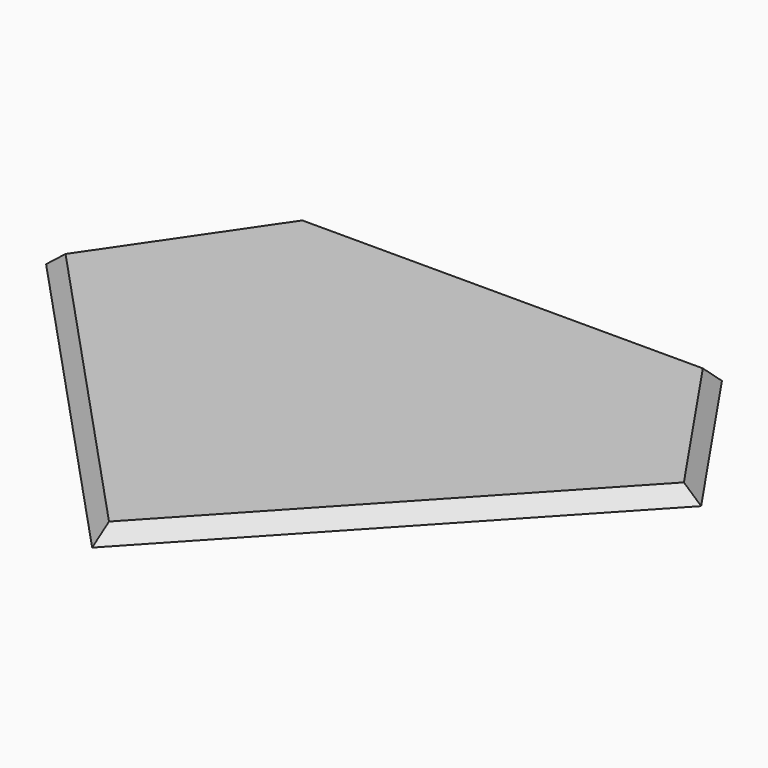
from build123d import *

# Parameters (mm, degrees)
F1_DEPTH    = 2.4268273264
F2_T1_DEPTH = 99.1532575298
F3_T1_DEPTH = 59.396472342
F4_T1_DEPTH = 59.396472342
F5_T1_DEPTH = 107.0840707021
F6_T1_DEPTH = 101.9910508867


# Not quite as in the source:
# - a fillet or chamfer that OpenCascade refuses, or shapes differently, is made with other operations: its cross-section is extruded or revolved along the edge and cut away or added


with BuildPart() as f1:
    # F0 (on Top) → F1 (new body)
    with BuildSketch(Plane.XY):
        Polygon((0, 32.5707793236), (-36.5124791861, 32.5707793236), (-58.7103962898, 0), (0, -63.0669593811), align=None)
        Polygon((36.5124791861, 32.5707793236), (0, 32.5707793236), (0, -63.0669593811), (58.7103962898, 0), align=None)
    extrude(amount=F1_DEPTH)

    # F2: chamfer of 5.08 on 1 edges, made by hand

    # F2_s2 → F2_t1 (cut)
    with BuildSketch(Plane.YZ.offset(-49.5766287649)):
        Polygon((32.5707793236, -2.6531726736), (27.4907793236, 2.4268273264), (32.5707793236, 2.4268273264), align=None)
    extrude(amount=F2_T1_DEPTH, mode=Mode.SUBTRACT)

    # F3: chamfer of 5.08 on 1 edges, made by hand

    # F3_s2 → F3_t1 (cut)
    with BuildSketch(Plane(origin=(7.4722902543, 10.964015938, 0), x_dir=(0, 0, 1), z_dir=(-0.5631734509, -0.8263387103, 0))):
        Polygon((-2.6531726736, 48.5146731522), (2.4268273264, 43.4346731522), (2.4268273264, 48.5146731522), align=None)
    extrude(amount=F3_T1_DEPTH, mode=Mode.SUBTRACT)

    # F4: chamfer of 5.08 on 1 edges, made by hand

    # F4_s2 → F4_t1 (cut)
    with BuildSketch(Plane(origin=(25.9782260477, -38.1175884143, 0), x_dir=(0, 0, 1), z_dir=(-0.5631734509, 0.8263387103, 0))):
        Polygon((-2.6531726736, 48.5146731522), (2.4268273264, 43.4346731522), (2.4268273264, 48.5146731522), align=None)
    extrude(amount=F4_T1_DEPTH, mode=Mode.SUBTRACT)

    # F5: chamfer of 5.08 on 1 edges, made by hand

    # F5_s2 → F5_t1 (cut)
    with BuildSketch(Plane(origin=(-40.354442867, -43.3489155239, 0), x_dir=(0, 0, 1), z_dir=(0.6813742779, 0.7319351703, 0))):
        Polygon((-2.6531726736, 42.9722039049), (2.4268273264, 37.8922039049), (2.4268273264, 42.9722039049), align=None)
    extrude(amount=F5_T1_DEPTH, mode=Mode.SUBTRACT)

    # F6: chamfer of 5.08 on 1 edges, made by hand

    # F6_s2 → F6_t1 (cut)
    with BuildSketch(Plane(origin=(-32.6098884775, 35.0296819984, 0), x_dir=(0, 0, 1), z_dir=(0.6813742779, -0.7319351703, 0))):
        Polygon((-2.6531726736, 42.9722039049), (2.4268273264, 37.8922039049), (2.4268273264, 42.9722039049), align=None)
    extrude(amount=F6_T1_DEPTH, mode=Mode.SUBTRACT)


solid = f1.part
